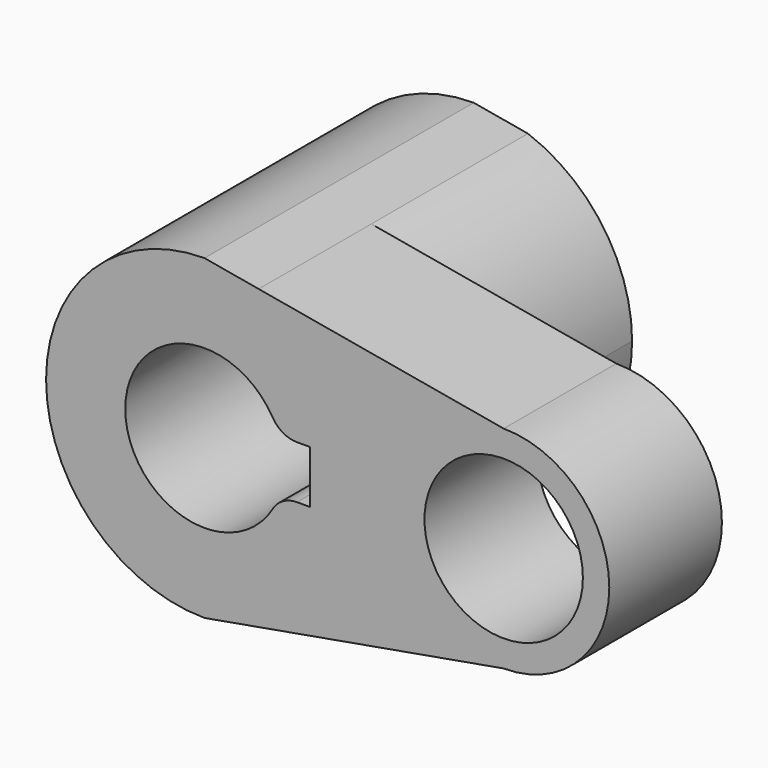
from build123d import *

# Parameters (mm, degrees)
F0_R     = 14.2875
F1_DEPTH = 25.4
F2_DEPTH = 35.306
F3_R     = 5.08


with BuildPart() as f1:
    # F0 (on Front) → F1 (new body)
    with BuildSketch(Plane.XZ):
        with BuildLine():
            Line((9.780704698, 26.8489932886), (0, 28.575))
            ThreePointArc((0, 28.575), (-28.575, 0), (0, -28.575))
            Line((0, -28.575), (9.7850073358, -26.8474255086))
            ThreePointArc((9.7850073358, -26.8474255086), (23.4108651017, -16.3848106547), (28.575, 0))
            ThreePointArc((28.575, 0), (23.4095521288, 16.3866864902), (9.780704698, 26.8489932886))
        make_face()
        with BuildLine():
            ThreePointArc((-13.4703841816, 4.7625), (0, 14.2875), (13.4703841816, 4.7625))
            Line((13.4703841816, 4.7625), (19.05, 4.7625))
            Line((19.05, 4.7625), (19.05, -4.7625))
            Line((19.05, -4.7625), (13.4703841816, -4.7625))
            ThreePointArc((13.4703841816, -4.7625), (0, -14.2875), (-13.4703841816, -4.7625))
            Line((-13.4703841816, -4.7625), (-19.05, -4.7625))
            Line((-19.05, -4.7625), (-19.05, 4.7625))
            Line((-19.05, 4.7625), (-13.4703841816, 4.7625))
        make_face(mode=Mode.SUBTRACT)
        with BuildLine():
            Line((53.975, 19.05), (9.780704698, 26.8489932886))
            ThreePointArc((9.780704698, 26.8489932886), (23.4095521288, 16.3866864902), (28.575, 0))
            ThreePointArc((28.575, 0), (23.4108651017, -16.3848106547), (9.7850073358, -26.8474255086))
            Line((9.7850073358, -26.8474255086), (53.949834283, -19.0499833776))
            ThreePointArc((53.949834283, -19.0499833776), (34.9250041556, 0.0125828612), (53.975, 19.05))
        make_face()
        with BuildLine():
            ThreePointArc((73.025, 0), (67.4453841816, 13.4703841816), (53.975, 19.05))
            ThreePointArc((53.975, 19.05), (34.9250041556, 0.0125828612), (53.949834283, -19.0499833776))
            ThreePointArc((53.949834283, -19.0499833776), (67.4364838166, -13.4792786697), (73.025, 0))
        make_face()
        with Locations((53.975, 0)):
            Circle(F0_R, mode=Mode.SUBTRACT)
        with BuildLine():
            ThreePointArc((-13.4703841816, -4.7625), (-14.2875, 0), (-13.4703841816, 4.7625))
            Line((-13.4703841816, 4.7625), (-19.05, 4.7625))
            Line((-19.05, 4.7625), (-19.05, -4.7625))
            Line((-19.05, -4.7625), (-13.4703841816, -4.7625))
        make_face()
    extrude(amount=F1_DEPTH)

    # F0 (on Front) → F2 (join)
    with BuildSketch(Plane.XZ):
        with BuildLine():
            Line((9.780704698, 26.8489932886), (0, 28.575))
            ThreePointArc((0, 28.575), (-28.575, 0), (0, -28.575))
            Line((0, -28.575), (9.7850073358, -26.8474255086))
            ThreePointArc((9.7850073358, -26.8474255086), (23.4108651017, -16.3848106547), (28.575, 0))
            ThreePointArc((28.575, 0), (23.4095521288, 16.3866864902), (9.780704698, 26.8489932886))
        make_face()
        with BuildLine():
            ThreePointArc((-13.4703841816, 4.7625), (0, 14.2875), (13.4703841816, 4.7625))
            Line((13.4703841816, 4.7625), (19.05, 4.7625))
            Line((19.05, 4.7625), (19.05, -4.7625))
            Line((19.05, -4.7625), (13.4703841816, -4.7625))
            ThreePointArc((13.4703841816, -4.7625), (0, -14.2875), (-13.4703841816, -4.7625))
            Line((-13.4703841816, -4.7625), (-19.05, -4.7625))
            Line((-19.05, -4.7625), (-19.05, 4.7625))
            Line((-19.05, 4.7625), (-13.4703841816, 4.7625))
        make_face(mode=Mode.SUBTRACT)
        with BuildLine():
            ThreePointArc((-13.4703841816, -4.7625), (-14.2875, 0), (-13.4703841816, 4.7625))
            Line((-13.4703841816, 4.7625), (-19.05, 4.7625))
            Line((-19.05, 4.7625), (-19.05, -4.7625))
            Line((-19.05, -4.7625), (-13.4703841816, -4.7625))
        make_face()
    extrude(amount=-F2_DEPTH)

    # F3
    f3_edges = [f1.edges().sort_by_distance(p)[0] for p in [
        (13.470384, 4.953, -4.7625),
        (13.470384, 4.953, 4.7625),
    ]]
    fillet(f3_edges, radius=F3_R)


solid = f1.part
